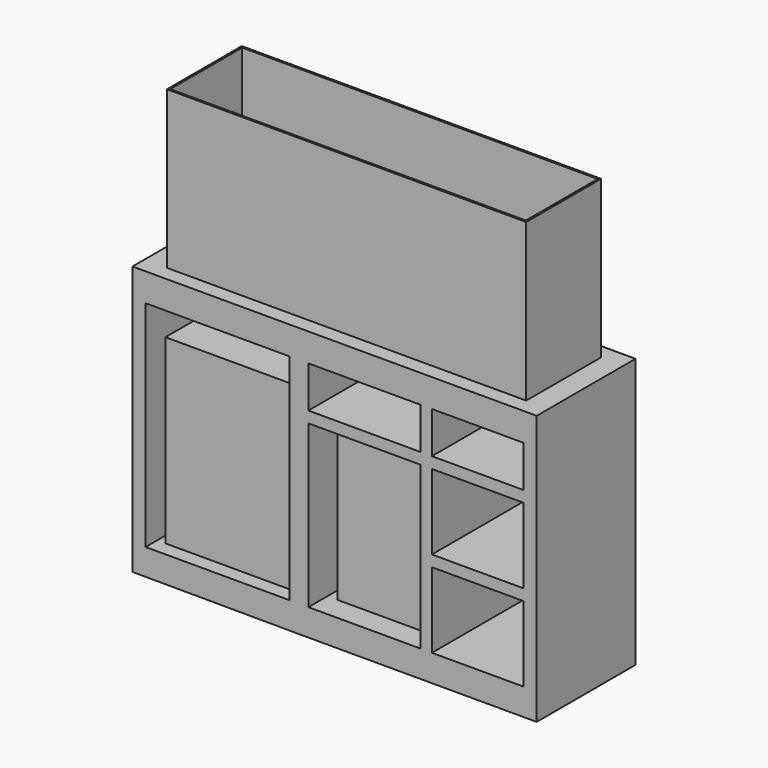
from build123d import *

# Parameters (mm, degrees)
F0_W           = 1219.2
F0_H           = 533.4
F1_DEPTH       = 317.5
F2_W           = 1206.5
F2_H           = 304.8
F3_DEPTH       = 527.05
F4_W           = 44.45
F4_H           = 728.299479103
F4_W_2         = 31.75
F4_H_2         = 90.850520897
F4_H_3         = 95.25
F5_DEPTH       = 368.3
F5_DEPTH_BACK  = 50.8
F8_W           = 425.45
F8_H           = 615.95
F9_DEPTH       = 158.75
F9_DEPTH_BACK  = 158.75
F10_W          = 304.8
F10_H          = 508
F11_DEPTH      = 127
F11_DEPTH_BACK = 127
F12_W          = 381
F12_H          = 38.1
F12_W_2        = 38.1
F12_H_2        = 140.987979103
F12_W_3        = 311.15
F13_DEPTH      = 419.1


with BuildPart() as f1:
    # F0 (on Front) → F1 (new body)
    with BuildSketch(Plane.XZ):
        with Locations((609.6, 266.7)):
            Rectangle(F0_W, F0_H)
    extrude(amount=F1_DEPTH)

    # F2 (on face) → F3 (cut)
    with BuildSketch(Plane.XY.offset(533.4)):
        with Locations((609.6, -158.75)):
            Rectangle(F2_W, F2_H)
    extrude(amount=-F3_DEPTH, mode=Mode.SUBTRACT)

    # F4 (on face) → F5 (join, two sides)
    with BuildSketch(Plane.XZ.offset(317.5)) as f5_sk:
        with Locations((-53.975, -459.3997395515)):
            Rectangle(F4_W, F4_H)
        Polygon((-31.75, -823.549479103), (-76.2, -823.549479103), (-76.2, -912.449479103), (457.2, -914.2904201743), (457.2, -823.549479103), align=None)
        with Locations((473.075, -459.3997395515)):
            Rectangle(F4_W_2, F4_H)
        with Locations((504.825, -459.3997395515)):
            Rectangle(F4_W_2, F4_H)
        Polygon((488.95, -823.549479103), (457.2, -823.549479103), (457.2, -914.2904201743), (488.95, -914.4), align=None)
        Polygon((520.7, -823.549479103), (488.95, -823.549479103), (488.95, -914.4), (1250.95, -914.4), (1250.95, -823.549479103), align=None)
        with Locations((1273.175, -868.9747395515)):
            Rectangle(F4_W, F4_H_2)
        with Locations((1273.175, -459.3997395515)):
            Rectangle(F4_W, F4_H)
        with Locations((1273.175, -47.625)):
            Rectangle(F4_W, F4_H_3)
        Polygon((1219.2, 0), (520.7, 0), (520.7, -95.25), (1250.95, -95.25), (1250.95, 0), align=None)
        Polygon((0, 0), (-31.75, 0), (-31.75, -95.25), (457.2, -95.25), (457.2, 0), align=None)
        with Locations((-53.975, -47.625)):
            Rectangle(F4_W, F4_H_3)
        with Locations((504.825, -47.625)):
            Rectangle(F4_W_2, F4_H_3)
        with Locations((473.075, -47.625)):
            Rectangle(F4_W_2, F4_H_3)
    extrude(amount=-F5_DEPTH)
    extrude(f5_sk.sketch, amount=F5_DEPTH_BACK)

    # F12 (on face) → F13 (join, through all)
    with BuildSketch(Plane.XZ.offset(368.3)):
        with Locations((711.2, -255.287979103)):
            Rectangle(F12_W, F12_H)
        with Locations((920.75, -165.7439895515)):
            Rectangle(F12_W_2, F12_H_2)
        with Locations((920.75, -255.287979103)):
            Rectangle(F12_W_2, F12_H)
        with Locations((1095.375, -255.287979103)):
            Rectangle(F12_W_3, F12_H)
        Polygon((939.8, -274.337979103), (901.7, -274.337979103), (901.7, -823.549479103), (939.8, -823.549479103), (939.8, -567.993729103), (939.8, -529.893729103), align=None)
        with Locations((1095.375, -548.943729103)):
            Rectangle(F12_W_3, F12_H)
    extrude(amount=-F13_DEPTH)


with BuildPart() as f9:
    # F8 (on face) → F9 (new body, two sides)
    with BuildSketch(Plane.XZ.offset(165.1)) as f9_sk:
        with Locations((212.725, -512.462979103)):
            Rectangle(F8_W, F8_H)
    extrude(amount=F9_DEPTH)
    extrude(f9_sk.sketch, amount=-F9_DEPTH_BACK)


with BuildPart() as f11:
    # F10 (on face) → F11 (new body, two sides)
    with BuildSketch(Plane.XZ.offset(165.1)) as f11_sk:
        with Locations((711.2, -566.437979103)):
            Rectangle(F10_W, F10_H)
    extrude(amount=F11_DEPTH)
    extrude(f11_sk.sketch, amount=-F11_DEPTH_BACK)


solid = Compound([f1.part, f9.part, f11.part])
